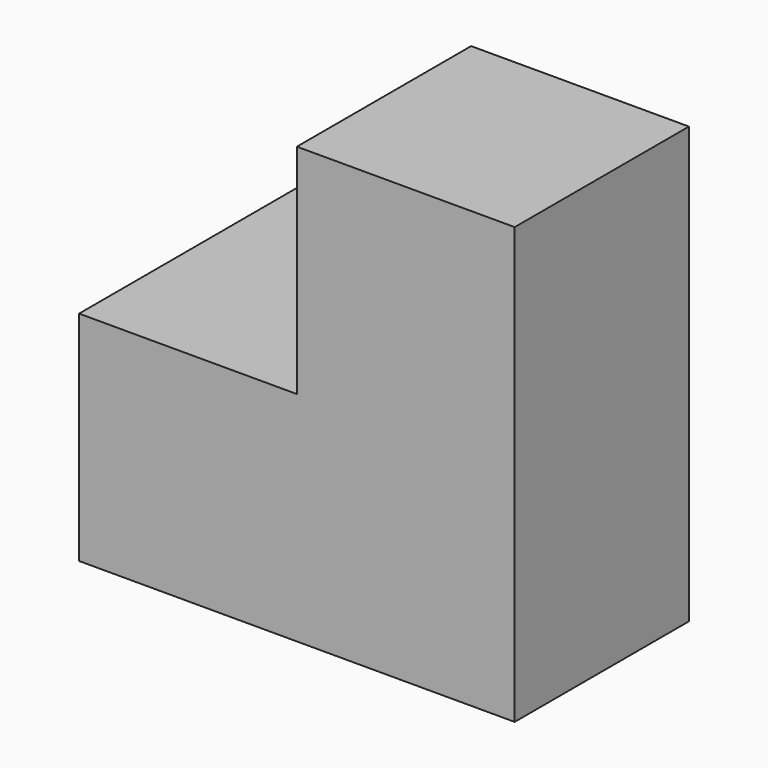
from build123d import *

# Parameters (mm, degrees)
F1_W     = 127
F1_H     = 127
F2_DEPTH = 127
F3_W     = 127
F3_H     = 127
F4_DEPTH = 127
F5_W     = 127
F5_H     = 127
F6_DEPTH = 127


# Not quite as in the source:
# - a variable given as a bare number and used for a length is read in inches; the dataset says mm whatever the document's units were


with BuildPart() as f2:
    # F1 (on Front) → F2 (new body, symmetric)
    with BuildSketch(Plane.XZ):
        Rectangle(F1_W, F1_H)
    extrude(amount=F2_DEPTH, both=True)

    # F3 (on face) → F4 (join)
    with BuildSketch(Plane.YZ.offset(63.5)):
        with Locations((-63.5, 0)):
            Rectangle(F3_W, F3_H)
    extrude(amount=F4_DEPTH)

    # F5 (on face) → F6 (join)
    with BuildSketch(Plane.XY.offset(63.5)):
        with Locations((127, -63.5)):
            Rectangle(F5_W, F5_H)
    extrude(amount=F6_DEPTH)


solid = f2.part
